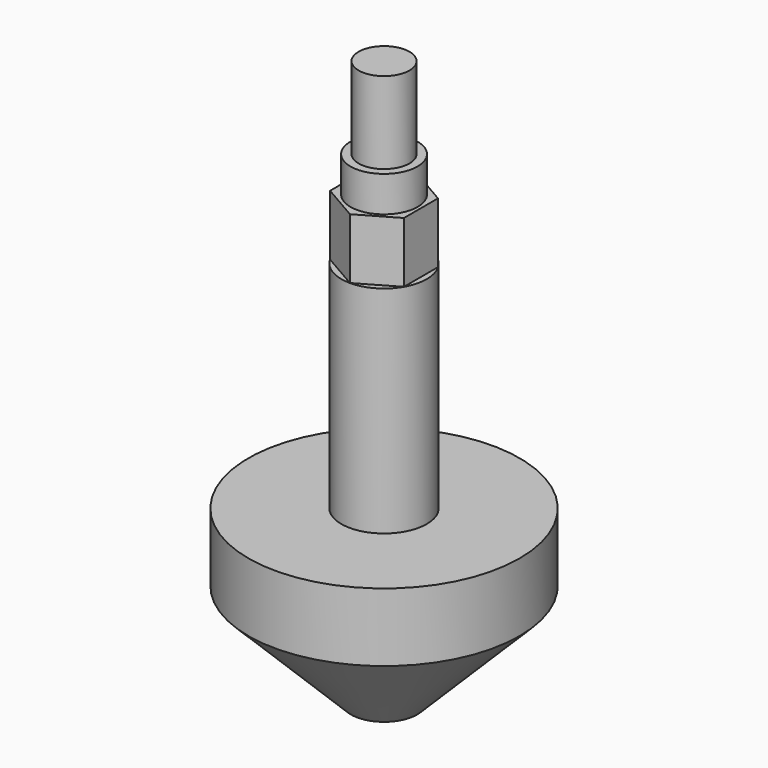
from build123d import *

# Parameters (mm, degrees)
F0_R     = 15.88
F0_R_2   = 10.66
F0_R_3   = 5
F0_R_4   = 3.93
F0_R_5   = 2.975
F1_DEPTH = 20
F2_DEPTH = 45.24
F3_DEPTH = 52.33
F4_DEPTH = 56.5
F5_DEPTH = 66.08
F7_SIZE  = 12


# Not quite as in the source:
# - a feature names something its author has since deleted; it is built from what else it names


with BuildPart() as f1:
    # F0 (on Top) → F1 (new body)
    with BuildSketch(Plane.XY):
        Circle(F0_R)
        Circle(F0_R_2, mode=Mode.SUBTRACT)
        Circle(F0_R_2)
        Circle(F0_R_3, mode=Mode.SUBTRACT)
        Circle(F0_R_3)
        Polygon((0, 4.9883063258), (4.32, 2.4941531629), (4.32, -2.4941531629), (0, -4.9883063258), (-4.32, -2.4941531629), (-4.32, 2.4941531629), align=None, mode=Mode.SUBTRACT)
        Polygon((4.32, -2.4941531629), (4.32, 2.4941531629), (0, 4.9883063258), (-4.32, 2.4941531629), (-4.32, -2.4941531629), (0, -4.9883063258), align=None)
        Circle(F0_R_4, mode=Mode.SUBTRACT)
        Circle(F0_R_4)
        Circle(F0_R_5, mode=Mode.SUBTRACT)
        Circle(F0_R_5)
    extrude(amount=F1_DEPTH)

    # F0 (on Top) → F2 (join)
    with BuildSketch(Plane.XY):
        Circle(F0_R_3)
        Polygon((0, 4.9883063258), (4.32, 2.4941531629), (4.32, -2.4941531629), (0, -4.9883063258), (-4.32, -2.4941531629), (-4.32, 2.4941531629), align=None, mode=Mode.SUBTRACT)
        Polygon((4.32, -2.4941531629), (4.32, 2.4941531629), (0, 4.9883063258), (-4.32, 2.4941531629), (-4.32, -2.4941531629), (0, -4.9883063258), align=None)
        Circle(F0_R_4, mode=Mode.SUBTRACT)
        Circle(F0_R_4)
        Circle(F0_R_5, mode=Mode.SUBTRACT)
        Circle(F0_R_5)
    extrude(amount=F2_DEPTH)

    # F0 (on Top) → F3 (join)
    with BuildSketch(Plane.XY):
        Polygon((4.32, -2.4941531629), (4.32, 2.4941531629), (0, 4.9883063258), (-4.32, 2.4941531629), (-4.32, -2.4941531629), (0, -4.9883063258), align=None)
        Circle(F0_R_4, mode=Mode.SUBTRACT)
        Circle(F0_R_4)
        Circle(F0_R_5, mode=Mode.SUBTRACT)
        Circle(F0_R_5)
    extrude(amount=F3_DEPTH)

    # F0 (on Top) → F4 (join)
    with BuildSketch(Plane.XY):
        Circle(F0_R_4)
        Circle(F0_R_5, mode=Mode.SUBTRACT)
        Circle(F0_R_5)
    extrude(amount=F4_DEPTH)

    # F0 (on Top) → F5 (join)
    with BuildSketch(Plane.XY):
        Circle(F0_R_5)
    extrude(amount=F5_DEPTH)

    # F7
    f7_edges = [f1.edges().sort_by_distance(p)[0] for p in [
        (-15.88, 0, 0),
    ]]
    chamfer(f7_edges, length=F7_SIZE)


solid = f1.part
